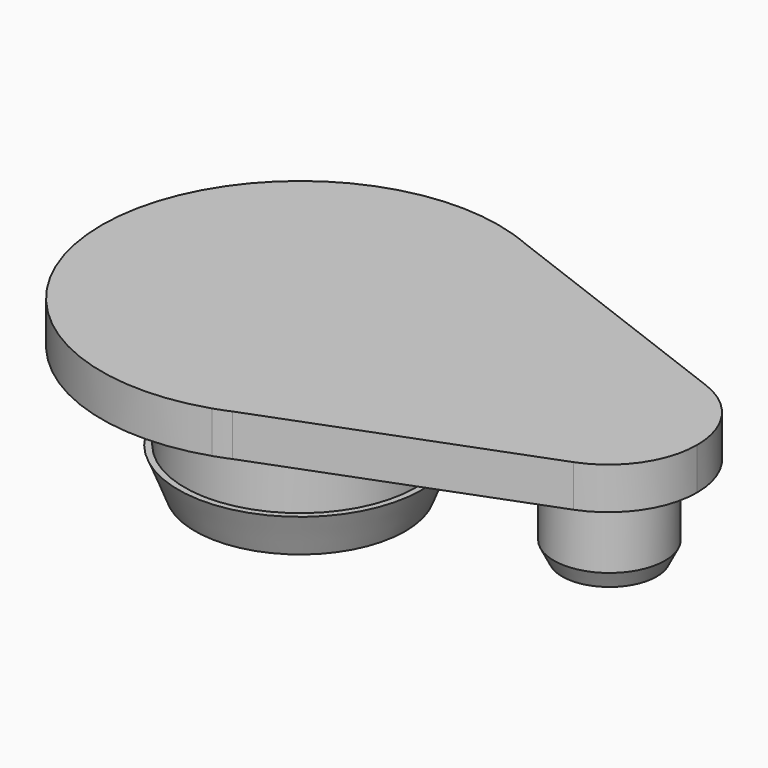
from build123d import *

# Parameters (mm, degrees)
F1_DEPTH = 2.5
F2_R     = 6.9
F2_R_2   = 4.95
F2_R_3   = 3.325
F2_R_4   = 1.15
F3_DEPTH = 5.2
F4_R     = 7.275
F4_R_2   = 4.95
F5_DEPTH = 2.5
F6_SIZE2 = 2.49999
F6_SIZE  = 0.99999
F7_SIZE2 = 1
F7_SIZE  = 0.5


# Not quite as in the source:
# - a fillet or chamfer is up to 0.001 mm smaller than in the source, because OpenCascade refuses the exact size


with BuildPart() as f1:
    # F0 (on Top) → F1 (new body)
    with BuildSketch(Plane.XY):
        with BuildLine():
            Line((4.6819136376, 10.8858708742), (3.7330328633, 11.2466424164))
            ThreePointArc((3.7330328633, 11.2466424164), (-11.85, 0), (3.7330328633, -11.2466424164))
            Line((3.7330328633, -11.2466424164), (4.6819136376, -10.8858708742))
            ThreePointArc((4.6819136376, -10.8858708742), (9.8970494746, -6.5169710523), (11.85, 0))
            ThreePointArc((11.85, 0), (9.8970494746, 6.5169710523), (4.6819136376, 10.8858708742))
        make_face()
        with BuildLine():
            ThreePointArc((4.6819136376, 10.8858708742), (4.2113382884, 11.0764222482), (3.7330328633, 11.2466424164))
            Line((3.7330328633, 11.2466424164), (4.6819136376, 10.8858708742))
        make_face()
        with BuildLine():
            Line((4.6819136376, -10.8858708742), (3.7330328633, -11.2466424164))
            ThreePointArc((3.7330328633, -11.2466424164), (4.2113382884, -11.0764222482), (4.6819136376, -10.8858708742))
        make_face()
        with BuildLine():
            Line((20.2835521459, 4.9540116384), (4.6819136376, 10.8858708742))
            ThreePointArc((4.6819136376, 10.8858708742), (9.8970494746, 6.5169710523), (11.85, 0))
            ThreePointArc((11.85, 0), (9.8970494746, -6.5169710523), (4.6819136376, -10.8858708742))
            Line((4.6819136376, -10.8858708742), (20.2835521459, -4.9540116384))
            ThreePointArc((20.2835521459, -4.9540116384), (13.1, 0), (20.2835521459, 4.9540116384))
        make_face()
        with BuildLine():
            ThreePointArc((23.7, 0), (22.7630738232, 3.0089178808), (20.2835521459, 4.9540116384))
            ThreePointArc((20.2835521459, 4.9540116384), (13.1, 0), (20.2835521459, -4.9540116384))
            ThreePointArc((20.2835521459, -4.9540116384), (22.7630738232, -3.0089178808), (23.7, 0))
        make_face()
    extrude(amount=F1_DEPTH)

    # F2 (on Top) → F3 (join)
    with BuildSketch(Plane.XY):
        Circle(F2_R)
        Circle(F2_R_2, mode=Mode.SUBTRACT)
        with Locations((18.464056775, 0)):
            Circle(F2_R_3)
        with Locations((18.464056775, 0)):
            Circle(F2_R_4, mode=Mode.SUBTRACT)
    extrude(amount=-F3_DEPTH)

    # F4 (on face) → F5 (join)
    with BuildSketch(Plane(origin=(0, 0, -5.2), x_dir=(1, 0, 0), z_dir=(0, 0, -1))):
        Circle(F4_R)
        Circle(F4_R_2, mode=Mode.SUBTRACT)
    extrude(amount=F5_DEPTH)

    # F6 (size 1 and 2.5 in the source; OpenCascade refuses exactly that, so slightly less here)
    f6_edges = [f1.edges().sort_by_distance(p)[0] for p in [
        (-7.275, 0, -7.7),
    ]]
    f6_side = f1.faces().sort_by_distance((-7.069232, 0, -7.7))[0]
    chamfer(f6_edges, length=F6_SIZE, length2=F6_SIZE2, reference=f6_side)

    # F7
    f7_edges = [f1.edges().sort_by_distance(p)[0] for p in [
        (15.139057, 0, -5.2),
    ]]
    f7_side = f1.faces().sort_by_distance((15.233102, 0, -5.2))[0]
    chamfer(f7_edges, length=F7_SIZE, length2=F7_SIZE2, reference=f7_side)


solid = f1.part
